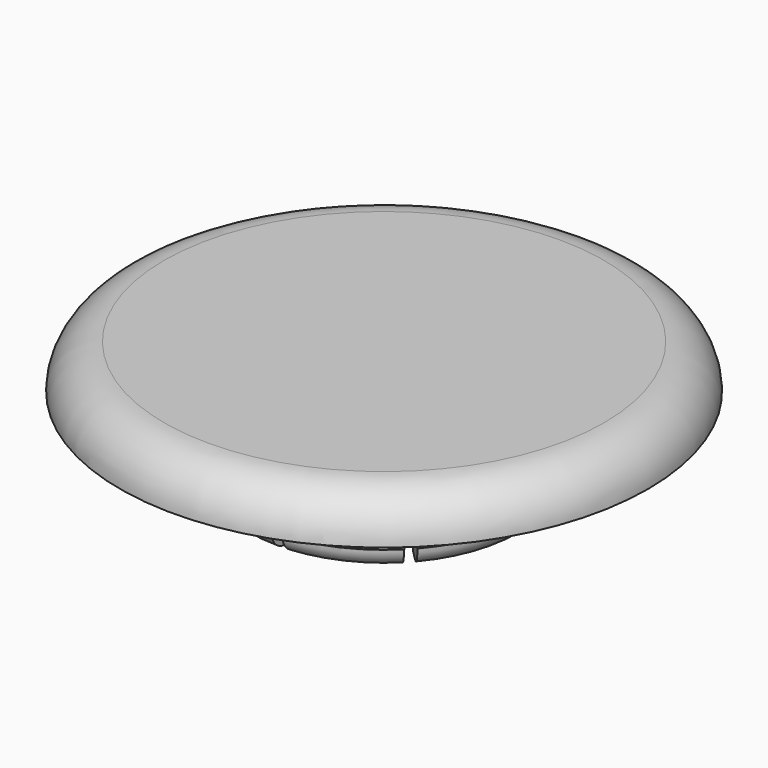
from build123d import *

# Parameters (mm, degrees)
F0_R      = 7.5
F0_R_2    = 4
F0_R_3    = 3.15
F1_DEPTH  = 1.25
F2_R      = 1.24999
F3_DEPTH  = 0.3
F4_R      = 4.15
F4_R_2    = 4
F5_DEPTH  = 0.3
F6_R      = 4
F7_DEPTH  = 0.3
F8_R      = 4.15
F9_DEPTH  = 0.3
F10_R     = 4
F11_DEPTH = 0.3
F12_R     = 4.15
F13_DEPTH = 0.3
F14_R     = 4
F15_DEPTH = 0.6
F16_R     = 0.5
F18_DEPTH = 2.25


# Not quite as in the source:
# - a fillet or chamfer is up to 0.001 mm smaller than in the source, because OpenCascade refuses the exact size


with BuildPart() as f1:
    # F0 (on Top) → F1 (new body)
    with BuildSketch(Plane.XY):
        Circle(F0_R)
        Circle(F0_R_2, mode=Mode.SUBTRACT)
        Circle(F0_R_2)
        Circle(F0_R_3, mode=Mode.SUBTRACT)
        Circle(F0_R_3)
    extrude(amount=F1_DEPTH)

    # F2 (radius 1.25 in the source; OpenCascade refuses exactly that, so slightly less here)
    f2_edges = [f1.edges().sort_by_distance(p)[0] for p in [
        (-7.5, 0, 1.25),
    ]]
    fillet(f2_edges, radius=F2_R)

    # F0 (on Top) → F3 (join)
    with BuildSketch(Plane.XY):
        Circle(F0_R_2)
        Circle(F0_R_3, mode=Mode.SUBTRACT)
        Circle(F0_R_3)
    extrude(amount=-F3_DEPTH)

    # F4 (on face) → F5 (join)
    with BuildSketch(Plane(origin=(0, 0, -0.3), x_dir=(1, 0, 0), z_dir=(0, 0, -1))):
        Circle(F4_R)
        Circle(F4_R_2, mode=Mode.SUBTRACT)
        Circle(F4_R_2)
    extrude(amount=F5_DEPTH)

    # F6 (on face) → F7 (join)
    with BuildSketch(Plane(origin=(0, 0, -0.6), x_dir=(1, 0, 0), z_dir=(0, 0, -1))):
        Circle(F6_R)
    extrude(amount=F7_DEPTH)

    # F8 (on face) → F9 (join)
    with BuildSketch(Plane(origin=(0, 0, -0.9), x_dir=(1, 0, 0), z_dir=(0, 0, -1))):
        Circle(F8_R)
    extrude(amount=F9_DEPTH)

    # F10 (on face) → F11 (join)
    with BuildSketch(Plane(origin=(0, 0, -1.2), x_dir=(1, 0, 0), z_dir=(0, 0, -1))):
        Circle(F10_R)
    extrude(amount=F11_DEPTH)

    # F12 (on face) → F13 (join)
    with BuildSketch(Plane(origin=(0, 0, -1.5), x_dir=(1, 0, 0), z_dir=(0, 0, -1))):
        Circle(F12_R)
    extrude(amount=F13_DEPTH)

    # F14 (on face) → F15 (join)
    with BuildSketch(Plane(origin=(0, 0, -1.8), x_dir=(1, 0, 0), z_dir=(0, 0, -1))):
        Circle(F14_R)
    extrude(amount=F15_DEPTH)

    # F16
    f16_edges = [f1.edges().sort_by_distance(p)[0] for p in [
        (-4, 0, -2.4),
    ]]
    fillet(f16_edges, radius=F16_R)

    # F17 (on face) → F18 (cut)
    with BuildSketch(Plane(origin=(0, 0, -2.4), x_dir=(1, 0, 0), z_dir=(0, 0, -1))):
        with BuildLine():
            Line((0.4242640687, 0), (3.15, 0))
            ThreePointArc((3.15, 0), (2.9643794171, 1.0653425138), (2.4293938592, 2.0051297905))
            Line((2.4293938592, 2.0051297905), (0.4242640687, 0))
        make_face()
        with BuildLine():
            Line((3.5, 0), (3.15, 0))
            ThreePointArc((3.15, 0), (3.1464183998, -0.1501707465), (3.1356817441, -0.3))
            Line((3.1356817441, -0.3), (3.4871191548, -0.3))
            ThreePointArc((3.4871191548, -0.3), (3.4967783059, -0.1501381998), (3.5, 0))
        make_face()
        with BuildLine():
            ThreePointArc((3.1356817441, -0.3), (3.1464183998, -0.1501707465), (3.15, 0))
            Line((3.15, 0), (0.4242640687, 0))
            Line((0.4242640687, 0), (0.2121320344, -0.2121320344))
            Line((0.2121320344, -0.2121320344), (0.3, -0.3))
            Line((0.3, -0.3), (3.1356817441, -0.3))
        make_face()
        with BuildLine():
            Line((0.4242640687, 0), (2.4293938592, 2.0051297905))
            ThreePointArc((2.4293938592, 2.0051297905), (2.3310405402, 2.1186670338), (2.2273863607, 2.2273863607))
            Line((2.2273863607, 2.2273863607), (0.3, 0.3))
            Line((0.3, 0.3), (0.3, 0))
            Line((0.3, 0), (0.4242640687, 0))
        make_face()
        with BuildLine():
            ThreePointArc((2.2273863607, 2.2273863607), (2.3310405402, 2.1186670338), (2.4293938592, 2.0051297905))
            Line((2.4293938592, 2.0051297905), (2.6778976355, 2.2536335668))
            ThreePointArc((2.6778976355, 2.2536335668), (2.5787593916, 2.3664319132), (2.4748737342, 2.4748737342))
            Line((2.4748737342, 2.4748737342), (2.2273863607, 2.2273863607))
        make_face()
        with BuildLine():
            ThreePointArc((2.2273863607, -2.2273863607), (2.8494437036, -1.342821872), (3.1356817441, -0.3))
            Line((3.1356817441, -0.3), (0.3, -0.3))
            Line((0.3, -0.3), (2.2273863607, -2.2273863607))
        make_face()
        with BuildLine():
            Line((6, 0), (3.5, 0))
            ThreePointArc((3.5, 0), (3.4967783059, -0.1501381998), (3.4871191548, -0.3))
            Line((3.4871191548, -0.3), (6, -0.3))
            Line((6, -0.3), (6, 0))
        make_face()
        Polygon((0.2121320344, -0.2121320344), (0.4242640687, 0), (0.3, 0), (0, 0), align=None)
        with BuildLine():
            Line((0.3, 0.3), (2.2273863607, 2.2273863607))
            ThreePointArc((2.2273863607, 2.2273863607), (1.342821872, 2.8494437036), (0.3, 3.1356817441))
            Line((0.3, 3.1356817441), (0.3, 0.3))
        make_face()
        with BuildLine():
            ThreePointArc((2.4748737342, 2.4748737342), (2.5787593916, 2.3664319132), (2.6778976355, 2.2536335668))
            Line((2.6778976355, 2.2536335668), (4.4547727215, 4.0305086528))
            Line((4.4547727215, 4.0305086528), (4.2426406871, 4.2426406871))
            Line((4.2426406871, 4.2426406871), (2.4748737342, 2.4748737342))
        make_face()
        with BuildLine():
            Line((2.4748737342, -2.4748737342), (2.2273863607, -2.2273863607))
            ThreePointArc((2.2273863607, -2.2273863607), (2.1186670338, -2.3310405402), (2.0051297905, -2.4293938592))
            Line((2.0051297905, -2.4293938592), (2.2536335668, -2.6778976355))
            ThreePointArc((2.2536335668, -2.6778976355), (2.3664319132, -2.5787593916), (2.4748737342, -2.4748737342))
        make_face()
        with BuildLine():
            ThreePointArc((2.0051297905, -2.4293938592), (2.1186670338, -2.3310405402), (2.2273863607, -2.2273863607))
            Line((2.2273863607, -2.2273863607), (0.3, -0.3))
            Line((0.3, -0.3), (0, -0.3))
            Line((0, -0.3), (0, -0.4242640687))
            Line((0, -0.4242640687), (2.0051297905, -2.4293938592))
        make_face()
        Polygon((0, -0.3), (0.3, -0.3), (0.2121320344, -0.2121320344), (0, 0), align=None)
        Polygon((0, 0), (0.3, 0), (0.3, 0.3), (0.2121320344, 0.2121320344), align=None)
        with BuildLine():
            Line((0.3, 0.3), (0.3, 3.1356817441))
            ThreePointArc((0.3, 3.1356817441), (0.1501707465, 3.1464183998), (0, 3.15))
            Line((0, 3.15), (0, 0.4242640687))
            Line((0, 0.4242640687), (0.2121320344, 0.2121320344))
            Line((0.2121320344, 0.2121320344), (0.3, 0.3))
        make_face()
        with BuildLine():
            ThreePointArc((0, 3.15), (0.1501707465, 3.1464183998), (0.3, 3.1356817441))
            Line((0.3, 3.1356817441), (0.3, 3.4871191548))
            ThreePointArc((0.3, 3.4871191548), (0.1501381998, 3.4967783059), (0, 3.5))
            Line((0, 3.5), (0, 3.15))
        make_face()
        with BuildLine():
            ThreePointArc((0, -3.15), (1.0653425138, -2.9643794171), (2.0051297905, -2.4293938592))
            Line((2.0051297905, -2.4293938592), (0, -0.4242640687))
            Line((0, -0.4242640687), (0, -3.15))
        make_face()
        with BuildLine():
            Line((4.2426406871, -4.2426406871), (2.4748737342, -2.4748737342))
            ThreePointArc((2.4748737342, -2.4748737342), (2.3664319132, -2.5787593916), (2.2536335668, -2.6778976355))
            Line((2.2536335668, -2.6778976355), (4.0305086528, -4.4547727215))
            Line((4.0305086528, -4.4547727215), (4.2426406871, -4.2426406871))
        make_face()
        Polygon((0, -0.4242640687), (0, -0.3), (0, 0), (-0.2121320344, -0.2121320344), align=None)
        Polygon((-0.2121320344, 0.2121320344), (0, 0), (0, 0.3), (-0.3, 0.3), align=None)
        Polygon((-0.3, 0), (0, 0), (-0.2121320344, 0.2121320344), (-0.4242640687, 0), align=None)
        Polygon((-0.2121320344, -0.2121320344), (0, 0), (-0.3, 0), (-0.3, -0.3), align=None)
        Polygon((0, 0.3), (0, 0), (0.2121320344, 0.2121320344), (0, 0.4242640687), align=None)
        with BuildLine():
            Line((0, 0.4242640687), (0, 3.15))
            ThreePointArc((0, 3.15), (-1.0653425138, 2.9643794171), (-2.0051297905, 2.4293938592))
            Line((-2.0051297905, 2.4293938592), (0, 0.4242640687))
        make_face()
        with BuildLine():
            ThreePointArc((0, 3.5), (0.1501381998, 3.4967783059), (0.3, 3.4871191548))
            Line((0.3, 3.4871191548), (0.3, 6))
            Line((0.3, 6), (0, 6))
            Line((0, 6), (0, 3.5))
        make_face()
        with BuildLine():
            Line((0, -3.5), (0, -3.15))
            ThreePointArc((0, -3.15), (-0.1501707465, -3.1464183998), (-0.3, -3.1356817441))
            Line((-0.3, -3.1356817441), (-0.3, -3.4871191548))
            ThreePointArc((-0.3, -3.4871191548), (-0.1501381998, -3.4967783059), (0, -3.5))
        make_face()
        with BuildLine():
            ThreePointArc((-0.3, -3.1356817441), (-0.1501707465, -3.1464183998), (0, -3.15))
            Line((0, -3.15), (0, -0.4242640687))
            Line((0, -0.4242640687), (-0.2121320344, -0.2121320344))
            Line((-0.2121320344, -0.2121320344), (-0.3, -0.3))
            Line((-0.3, -0.3), (-0.3, -3.1356817441))
        make_face()
        with BuildLine():
            Line((-0.3, 0.3), (0, 0.3))
            Line((0, 0.3), (0, 0.4242640687))
            Line((0, 0.4242640687), (-2.0051297905, 2.4293938592))
            ThreePointArc((-2.0051297905, 2.4293938592), (-2.1186670338, 2.3310405402), (-2.2273863607, 2.2273863607))
            Line((-2.2273863607, 2.2273863607), (-0.3, 0.3))
        make_face()
        with BuildLine():
            Line((-0.4242640687, 0), (-0.2121320344, 0.2121320344))
            Line((-0.2121320344, 0.2121320344), (-0.3, 0.3))
            Line((-0.3, 0.3), (-3.1356817441, 0.3))
            ThreePointArc((-3.1356817441, 0.3), (-3.1464183998, 0.1501707465), (-3.15, 0))
            Line((-3.15, 0), (-0.4242640687, 0))
        make_face()
        with BuildLine():
            Line((-0.3, -0.3), (-0.3, 0))
            Line((-0.3, 0), (-0.4242640687, 0))
            Line((-0.4242640687, 0), (-2.4293938592, -2.0051297905))
            ThreePointArc((-2.4293938592, -2.0051297905), (-2.3310405402, -2.1186670338), (-2.2273863607, -2.2273863607))
            Line((-2.2273863607, -2.2273863607), (-0.3, -0.3))
        make_face()
        with BuildLine():
            ThreePointArc((-2.2273863607, 2.2273863607), (-2.1186670338, 2.3310405402), (-2.0051297905, 2.4293938592))
            Line((-2.0051297905, 2.4293938592), (-2.2536335668, 2.6778976355))
            ThreePointArc((-2.2536335668, 2.6778976355), (-2.3664319132, 2.5787593916), (-2.4748737342, 2.4748737342))
            Line((-2.4748737342, 2.4748737342), (-2.2273863607, 2.2273863607))
        make_face()
        with BuildLine():
            ThreePointArc((-2.2273863607, -2.2273863607), (-1.342821872, -2.8494437036), (-0.3, -3.1356817441))
            Line((-0.3, -3.1356817441), (-0.3, -0.3))
            Line((-0.3, -0.3), (-2.2273863607, -2.2273863607))
        make_face()
        with BuildLine():
            Line((0, -6), (0, -3.5))
            ThreePointArc((0, -3.5), (-0.1501381998, -3.4967783059), (-0.3, -3.4871191548))
            Line((-0.3, -3.4871191548), (-0.3, -6))
            Line((-0.3, -6), (0, -6))
        make_face()
        with BuildLine():
            Line((-3.1356817441, 0.3), (-0.3, 0.3))
            Line((-0.3, 0.3), (-2.2273863607, 2.2273863607))
            ThreePointArc((-2.2273863607, 2.2273863607), (-2.8494437036, 1.342821872), (-3.1356817441, 0.3))
        make_face()
        with BuildLine():
            Line((-2.4293938592, -2.0051297905), (-0.4242640687, 0))
            Line((-0.4242640687, 0), (-3.15, 0))
            ThreePointArc((-3.15, 0), (-2.9643794171, -1.0653425138), (-2.4293938592, -2.0051297905))
        make_face()
        with BuildLine():
            ThreePointArc((-2.4748737342, 2.4748737342), (-2.3664319132, 2.5787593916), (-2.2536335668, 2.6778976355))
            Line((-2.2536335668, 2.6778976355), (-4.0305086528, 4.4547727215))
            Line((-4.0305086528, 4.4547727215), (-4.2426406871, 4.2426406871))
            Line((-4.2426406871, 4.2426406871), (-2.4748737342, 2.4748737342))
        make_face()
        with BuildLine():
            Line((-2.4748737342, -2.4748737342), (-2.2273863607, -2.2273863607))
            ThreePointArc((-2.2273863607, -2.2273863607), (-2.3310405402, -2.1186670338), (-2.4293938592, -2.0051297905))
            Line((-2.4293938592, -2.0051297905), (-2.6778976355, -2.2536335668))
            ThreePointArc((-2.6778976355, -2.2536335668), (-2.5787593916, -2.3664319132), (-2.4748737342, -2.4748737342))
        make_face()
        with BuildLine():
            ThreePointArc((-3.15, 0), (-3.1464183998, 0.1501707465), (-3.1356817441, 0.3))
            Line((-3.1356817441, 0.3), (-3.4871191548, 0.3))
            ThreePointArc((-3.4871191548, 0.3), (-3.4967783059, 0.1501381998), (-3.5, 0))
            Line((-3.5, 0), (-3.15, 0))
        make_face()
        with BuildLine():
            Line((-4.2426406871, -4.2426406871), (-2.4748737342, -2.4748737342))
            ThreePointArc((-2.4748737342, -2.4748737342), (-2.5787593916, -2.3664319132), (-2.6778976355, -2.2536335668))
            Line((-2.6778976355, -2.2536335668), (-4.4547727215, -4.0305086528))
            Line((-4.4547727215, -4.0305086528), (-4.2426406871, -4.2426406871))
        make_face()
        with BuildLine():
            ThreePointArc((-3.5, 0), (-3.4967783059, 0.1501381998), (-3.4871191548, 0.3))
            Line((-3.4871191548, 0.3), (-6, 0.3))
            Line((-6, 0.3), (-6, 0))
            Line((-6, 0), (-3.5, 0))
        make_face()
    extrude(amount=-F18_DEPTH, mode=Mode.SUBTRACT)


solid = f1.part
